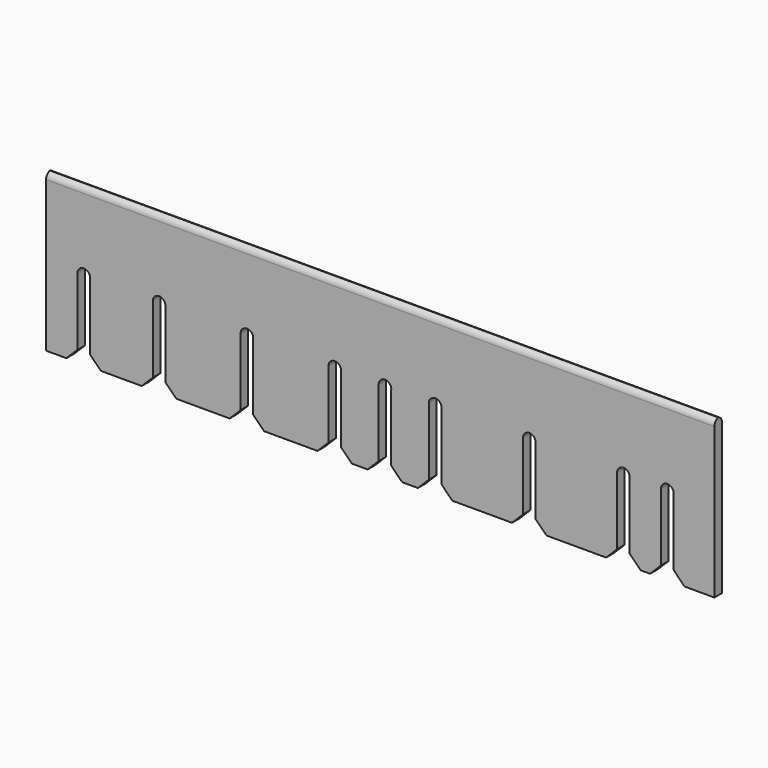
from build123d import *

# Parameters (mm, degrees)
F1_DEPTH    = 3
F2_SIZE     = 3.5
F3_T1_DEPTH = 223


# Not quite as in the source:
# - a fillet or chamfer that OpenCascade refuses, or shapes differently, is made with other operations: its cross-section is extruded or revolved along the edge and cut away or added


with BuildPart() as f1:
    # F0 (on Front) → F1 (new body)
    with BuildSketch(Plane.XZ):
        with BuildLine():
            Line((130.4753928185, 16.1237554376), (-82.5246071815, 16.1237554376))
            Line((-82.5246071815, 16.1237554376), (-82.5246071815, -33.8762445624))
            Line((-82.5246071815, -33.8762445624), (-72.5246071815, -33.8762445624))
            Line((-72.5246071815, -33.8762445624), (-72.5246071815, -8.8762445624))
            ThreePointArc((-72.5246071815, -8.8762445624), (-70.3837107757, -6.871899239), (-68.5246071815, -9.1400640085))
            Line((-68.5246071815, -9.1400640085), (-68.5246071815, -33.8762445624))
            Line((-68.5246071815, -33.8762445624), (-48.5246071815, -33.8762445624))
            Line((-48.5246071815, -33.8762445624), (-48.5246071815, -8.8762445624))
            ThreePointArc((-48.5246071815, -8.8762445624), (-46.3837107899, -6.8718992399), (-44.5246071815, -9.1400639837))
            Line((-44.5246071815, -9.1400639837), (-44.5246071815, -33.8762445624))
            Line((-44.5246071815, -33.8762445624), (-20.5246071815, -33.8762445624))
            Line((-20.5246071815, -33.8762445624), (-20.5246071815, -8.8762445624))
            ThreePointArc((-20.5246071815, -8.8762445624), (-18.3837111079, -6.8718992583), (-16.5246071815, -9.1400634249))
            Line((-16.5246071815, -9.1400634249), (-16.5246071815, -33.8762445624))
            Line((-16.5246071815, -33.8762445624), (7.4753928185, -33.8762445624))
            Line((7.4753928185, -33.8762445624), (7.4753928185, -8.8762445624))
            ThreePointArc((7.4753928185, -8.8762445624), (9.6162888921, -6.8718992583), (11.4753928185, -9.1400634249))
            Line((11.4753928185, -9.1400634249), (11.4753928185, -33.8762445624))
            Line((11.4753928185, -33.8762445624), (23.4753928185, -33.8762445624))
            Line((23.4753928185, -33.8762445624), (23.4753928185, -8.8762445624))
            ThreePointArc((23.4753928185, -8.8762445624), (25.6162892101, -6.8718992399), (27.4753928185, -9.1400639837))
            Line((27.4753928185, -9.1400639837), (27.4753928185, -33.8762445624))
            Line((27.4753928185, -33.8762445624), (39.4753928185, -33.8762445624))
            Line((39.4753928185, -33.8762445624), (39.4753928185, -8.8762445624))
            ThreePointArc((39.4753928185, -8.8762445624), (41.6162892243, -6.871899239), (43.4753928185, -9.1400640085))
            Line((43.4753928185, -9.1400640085), (43.4753928185, -33.8762445624))
            Line((43.4753928185, -33.8762445624), (69.4753928185, -33.8762445624))
            Line((69.4753928185, -33.8762445624), (69.4753928185, -8.8762445624))
            ThreePointArc((69.4753928185, -8.8762445624), (71.6162892243, -6.871899239), (73.4753928185, -9.1400640085))
            Line((73.4753928185, -9.1400640085), (73.4753928185, -33.8762445624))
            Line((73.4753928185, -33.8762445624), (99.4753928185, -33.8762445624))
            Line((99.4753928185, -33.8762445624), (99.4753928185, -8.8762445624))
            ThreePointArc((99.4753928185, -8.8762445624), (101.6162892243, -6.871899239), (103.4753928185, -9.1400640085))
            Line((103.4753928185, -9.1400640085), (103.4753928185, -33.8762445624))
            Line((103.4753928185, -33.8762445624), (113.4753928185, -33.8762445624))
            Line((113.4753928185, -33.8762445624), (113.4753928185, -8.8762445624))
            ThreePointArc((113.4753928185, -8.8762445624), (115.6162892243, -6.871899239), (117.4753928185, -9.1400640085))
            Line((117.4753928185, -9.1400640085), (117.4753928185, -33.8762445624))
            Line((117.4753928185, -33.8762445624), (130.4753928185, -33.8762445624))
            Line((130.4753928185, -33.8762445624), (130.4753928185, 16.1237554376))
        make_face()
    extrude(amount=F1_DEPTH)

    # F2
    f2_edges = [f1.edges().sort_by_distance(p)[0] for p in [
        (-72.524607, -1.5, -33.876245),
        (-48.524607, -1.5, -33.876245),
        (-20.524607, -1.5, -33.876245),
        (7.475393, -1.5, -33.876245),
        (23.475393, -1.5, -33.876245),
        (39.475393, -1.5, -33.876245),
        (69.475393, -1.5, -33.876245),
        (99.475393, -1.5, -33.876245),
        (113.475393, -1.5, -33.876245),
        (103.475393, -1.5, -33.876245),
        (117.475393, -1.5, -33.876245),
        (73.475393, -1.5, -33.876245),
        (43.475393, -1.5, -33.876245),
        (27.475393, -1.5, -33.876245),
        (11.475393, -1.5, -33.876245),
        (-16.524607, -1.5, -33.876245),
        (-44.524607, -1.5, -33.876245),
        (-68.524607, -1.5, -33.876245),
    ]]
    chamfer(f2_edges, length=F2_SIZE)

    # F3: fillet of radius 2 on 2 edges, made by hand

    # F3_s2 → F3_t1 (cut)
    with BuildSketch(Plane.YZ.offset(-87.5246071815)):
        with BuildLine():
            ThreePointArc((-3, 14.1237554376), (-2.4142135624, 15.537969), (-1, 16.1237554376))
            Line((-1, 16.1237554376), (-3, 16.1237554376))
            Line((-3, 16.1237554376), (-3, 14.1237554376))
        make_face()
        with BuildLine():
            ThreePointArc((0, 14.1237554376), (-0.5857864376, 15.537969), (-2, 16.1237554376))
            Line((-2, 16.1237554376), (0, 16.1237554376))
            Line((0, 16.1237554376), (0, 14.1237554376))
        make_face()
    extrude(amount=F3_T1_DEPTH, mode=Mode.SUBTRACT)


solid = f1.part
